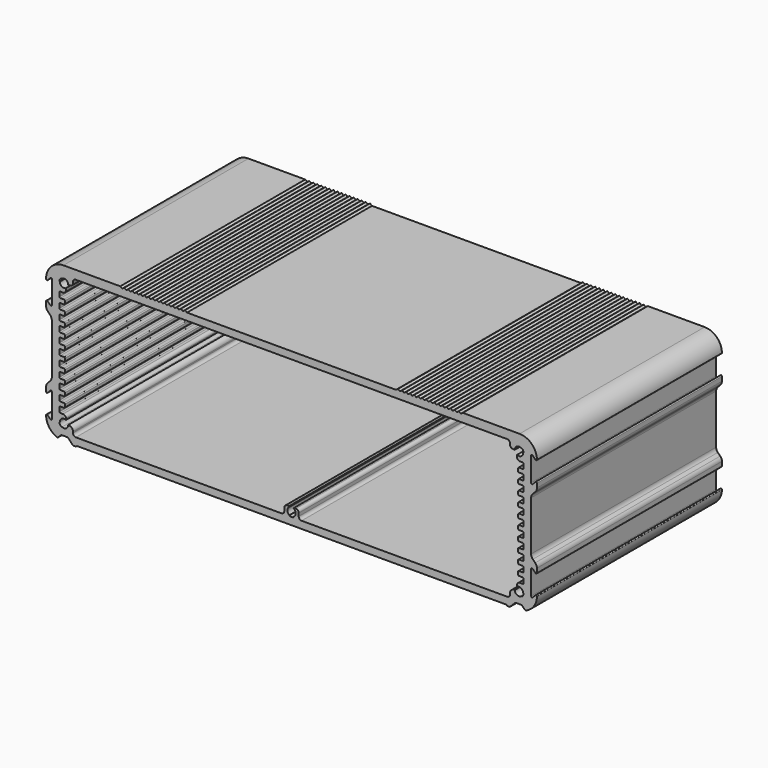
from build123d import *

# Parameters (mm, degrees)
F1_DEPTH = 80


# Not quite as in the source:
# - ends of sketch curves that miss each other by under 0.0002 mm in the source are joined


with BuildPart() as f1:
    # F0 (on Front) → F1 (new body)
    with BuildSketch(Plane.XZ):
        with BuildLine():
            Line((36.15, 26.4), (-36.15, 26.4))
            Line((-36.15, 26.4), (-36.85, 26.9))
            Line((-36.85, 26.9), (-37.55, 26.4))
            Line((-37.55, 26.4), (-38.25, 26.9))
            Line((-38.25, 26.9), (-38.95, 26.4))
            Line((-38.95, 26.4), (-39.65, 26.9))
            Line((-39.65, 26.9), (-40.35, 26.4))
            Line((-40.35, 26.4), (-41.05, 26.9))
            Line((-41.05, 26.9), (-41.75, 26.4))
            Line((-41.75, 26.4), (-42.45, 26.9))
            Line((-42.45, 26.9), (-43.15, 26.4))
            Line((-43.15, 26.4), (-43.85, 26.9))
            Line((-43.85, 26.9), (-44.55, 26.4))
            Line((-44.55, 26.4), (-45.25, 26.9))
            Line((-45.25, 26.9), (-45.95, 26.4))
            Line((-45.95, 26.4), (-46.65, 26.9))
            Line((-46.65, 26.9), (-47.35, 26.4))
            Line((-47.35, 26.4), (-48.05, 26.9))
            Line((-48.05, 26.9), (-48.75, 26.4))
            Line((-48.75, 26.4), (-49.45, 26.9))
            Line((-49.45, 26.9), (-50.15, 26.4))
            Line((-50.15, 26.4), (-50.85, 26.9))
            Line((-50.85, 26.9), (-51.55, 26.4))
            Line((-51.55, 26.4), (-52.25, 26.9))
            Line((-52.25, 26.9), (-52.95, 26.4))
            Line((-52.95, 26.4), (-53.65, 26.9))
            Line((-53.65, 26.9), (-54.35, 26.4))
            Line((-54.35, 26.4), (-55.05, 26.9))
            Line((-55.05, 26.9), (-55.75, 26.4))
            Line((-55.75, 26.4), (-56.45, 26.9))
            Line((-56.45, 26.9), (-57.15, 26.4))
            Line((-57.15, 26.4), (-57.85, 26.9))
            Line((-57.85, 26.9), (-58.55, 26.4))
            Line((-58.55, 26.4), (-59.25, 26.9))
            Line((-59.25, 26.9), (-78.9, 26.9))
            ThreePointArc((-78.9, 26.9), (-83.1426406871, 25.1426406871), (-84.9, 20.9))
            Line((-84.9, 20.9), (-84.9, 20.799264))
            ThreePointArc((-84.9, 20.799264), (-84.7148050297, 20.5221001402), (-84.3878679656, 20.5871319656))
            Line((-84.3878679656, 20.5871319656), (-83.412132, 21.562868))
            ThreePointArc((-83.412132, 21.562868), (-83.0851949703, 21.6278998598), (-82.9, 21.350736))
            Line((-82.9, 21.350736), (-82.9, 13.449264))
            ThreePointArc((-82.9, 13.449264), (-83.0851949703, 13.1721001402), (-83.4121320344, 13.2371319656))
            Line((-83.4121320344, 13.2371319656), (-84.387868, 14.212868))
            ThreePointArc((-84.387868, 14.212868), (-84.7148050297, 14.2778998598), (-84.9, 14.000736))
            Line((-84.9, 14.000736), (-84.9, 12.553427))
            ThreePointArc((-84.9, 12.553427), (-84.7477592003, 11.7880604619), (-84.3142140624, 11.1392139376))
            Line((-84.3142140624, 11.1392139376), (-83.485786, 10.310786))
            ThreePointArc((-83.485786, 10.310786), (-83.0497841884, 9.5556126224), (-82.9000002184, 8.6965730006))
            Line((-82.9000002184, 8.6965730006), (-82.9, -8.396573))
            ThreePointArc((-82.9, -8.396573), (-83.0522407997, -9.1619395381), (-83.4857859376, -9.8107860624))
            Line((-83.4857859376, -9.8107860624), (-84.314214, -10.639214))
            ThreePointArc((-84.314214, -10.639214), (-84.7477592003, -11.2880604619), (-84.9, -12.053427))
            Line((-84.9, -12.053427), (-84.9, -13.500736))
            ThreePointArc((-84.9, -13.500736), (-84.7148050297, -13.7778998598), (-84.3878679656, -13.7128680344))
            Line((-84.3878679656, -13.7128680344), (-83.412132, -12.737132))
            ThreePointArc((-83.412132, -12.737132), (-83.0851949703, -12.6721001402), (-82.9, -12.949264))
            Line((-82.9, -12.949264), (-82.9, -21.250736))
            ThreePointArc((-82.9, -21.250736), (-83.0851949703, -21.5278998598), (-83.4121320344, -21.4628680344))
            Line((-83.4121320344, -21.4628680344), (-84.387868, -20.487132))
            ThreePointArc((-84.387868, -20.487132), (-84.7115889033, -20.4049990304), (-84.8994513764, -20.6811310051))
            ThreePointArc((-84.8994513764, -20.6811310051), (-83.8330713991, -24.0153779543), (-81.0874780686, -26.1870331751))
            ThreePointArc((-81.0874780686, -26.1870331751), (-80.9167083168, -26.2013314216), (-80.7659719656, -26.1198130344))
            Line((-80.7659719656, -26.1198130344), (-79.734027, -25.087868))
            ThreePointArc((-79.734027, -25.087868), (-79.6367000297, -25.0228361402), (-79.521895, -25))
            Line((-79.521895, -25), (-77.575713, -25))
            ThreePointArc((-77.575713, -25), (-77.4609079703, -25.0228361402), (-77.3635809656, -25.0878679656))
            Line((-77.3635809656, -25.0878679656), (-75.551449, -26.9))
            Line((-75.551449, -26.9), (-74.551449, -26.9))
            Line((-74.551449, -26.9), (-74.251449, -26.6))
            Line((-74.251449, -26.6), (74.251449, -26.6))
            Line((74.251449, -26.6), (74.551449, -26.9))
            Line((74.551449, -26.9), (75.551449, -26.9))
            Line((75.551449, -26.9), (77.363581, -25.087868))
            ThreePointArc((77.363581, -25.087868), (77.4609079703, -25.0228361402), (77.575713, -25))
            Line((77.575713, -25), (79.521895, -25))
            ThreePointArc((79.521895, -25), (79.6367000297, -25.0228361402), (79.7340270344, -25.0878679656))
            Line((79.7340270344, -25.0878679656), (80.765972, -26.119813))
            ThreePointArc((80.765972, -26.119813), (80.9167083168, -26.2013314216), (81.0874778713, -26.1870326713))
            ThreePointArc((81.0874778713, -26.1870326713), (83.8330713991, -24.0153779543), (84.8994514549, -20.6811310062))
            ThreePointArc((84.8994514549, -20.6811310062), (84.7115889033, -20.4049990304), (84.3878677463, -20.4871317813))
            Line((84.3878677463, -20.4871317813), (83.412132, -21.462868))
            ThreePointArc((83.412132, -21.462868), (83.0851949703, -21.5278998598), (82.9, -21.250736))
            Line((82.9, -21.250736), (82.9, -12.949264))
            ThreePointArc((82.9, -12.949264), (83.0851949703, -12.6721001402), (83.4121320344, -12.7371319656))
            Line((83.4121320344, -12.7371319656), (84.387868, -13.712868))
            ThreePointArc((84.387868, -13.712868), (84.7148050297, -13.7778998598), (84.9, -13.500736))
            Line((84.9, -13.500736), (84.9, -12.053427))
            ThreePointArc((84.9, -12.053427), (84.7477592003, -11.2880604619), (84.3142140624, -10.6392139376))
            Line((84.3142140624, -10.6392139376), (83.485786, -9.810786))
            ThreePointArc((83.485786, -9.810786), (83.0522407997, -9.1619395381), (82.9, -8.396573))
            Line((82.9, -8.396573), (82.9, 8.696573))
            ThreePointArc((82.9, 8.696573), (83.0522407997, 9.4619395381), (83.4857859376, 10.1107860624))
            Line((83.4857859376, 10.1107860624), (84.314214, 10.939214))
            ThreePointArc((84.314214, 10.939214), (84.7477592003, 11.5880604619), (84.9, 12.353427))
            Line((84.9, 12.353427), (84.9, 13.800736))
            ThreePointArc((84.9, 13.800736), (84.7148050297, 14.0778998598), (84.3878679656, 14.0128680344))
            Line((84.3878679656, 14.0128680344), (83.412132, 13.037132))
            ThreePointArc((83.412132, 13.037132), (83.0851949703, 12.9721001402), (82.9, 13.249264))
            Line((82.9, 13.249264), (82.9, 21.550736))
            ThreePointArc((82.9, 21.550736), (83.0851949703, 21.8278998598), (83.4121320344, 21.7628680344))
            Line((83.4121320344, 21.7628680344), (84.387868, 20.787132))
            ThreePointArc((84.387868, 20.787132), (84.7063723422, 20.7187556671), (84.8994514873, 20.9811309705))
            ThreePointArc((84.8994514873, 20.9811309705), (83.1138589181, 25.171228514), (78.9, 26.9))
            Line((78.9, 26.9), (59.25, 26.9))
            Line((59.25, 26.9), (58.55, 26.4))
            Line((58.55, 26.4), (57.85, 26.9))
            Line((57.85, 26.9), (57.15, 26.4))
            Line((57.15, 26.4), (56.45, 26.9))
            Line((56.45, 26.9), (55.75, 26.4))
            Line((55.75, 26.4), (55.05, 26.9))
            Line((55.05, 26.9), (54.35, 26.4))
            Line((54.35, 26.4), (53.65, 26.9))
            Line((53.65, 26.9), (52.95, 26.4))
            Line((52.95, 26.4), (52.25, 26.9))
            Line((52.25, 26.9), (51.55, 26.4))
            Line((51.55, 26.4), (50.85, 26.9))
            Line((50.85, 26.9), (50.15, 26.4))
            Line((50.15, 26.4), (49.45, 26.9))
            Line((49.45, 26.9), (48.75, 26.4))
            Line((48.75, 26.4), (48.05, 26.9))
            Line((48.05, 26.9), (47.35, 26.4))
            Line((47.35, 26.4), (46.65, 26.9))
            Line((46.65, 26.9), (45.95, 26.4))
            Line((45.95, 26.4), (45.25, 26.9))
            Line((45.25, 26.9), (44.55, 26.4))
            Line((44.55, 26.4), (43.85, 26.9))
            Line((43.85, 26.9), (43.15, 26.4))
            Line((43.15, 26.4), (42.45, 26.9))
            Line((42.45, 26.9), (41.75, 26.4))
            Line((41.75, 26.4), (41.05, 26.9))
            Line((41.05, 26.9), (40.35, 26.4))
            Line((40.35, 26.4), (39.65, 26.9))
            Line((39.65, 26.9), (38.95, 26.4))
            Line((38.95, 26.4), (38.25, 26.9))
            Line((38.25, 26.9), (37.55, 26.4))
            Line((37.55, 26.4), (36.85, 26.9))
            Line((36.85, 26.9), (36.15, 26.4))
        make_face()
        with BuildLine():
            ThreePointArc((-75.6, 22.9), (-75.3071067812, 23.6071067812), (-74.6, 23.9))
            Line((-74.6, 23.9), (74.6, 23.9))
            ThreePointArc((74.6, 23.9), (75.3071067812, 23.6071067812), (75.6, 22.9))
            Line((75.6, 22.9), (75.6, 22.5))
            ThreePointArc((75.6, 22.5), (75.8928932188, 21.7928932188), (76.6, 21.5))
            Line((76.6, 21.5), (77.25, 21.5))
            ThreePointArc((77.25, 21.5), (78.0928837979, 22.8167801324), (79.6415998857, 22.6026738662))
            Line((79.6415998857, 22.6026738662), (79.726192, 22.727571))
            ThreePointArc((79.726192, 22.727571), (80.1494666284, 22.1775296991), (80.3, 21.5))
            Line((80.3, 21.5), (80.15, 21.5))
            ThreePointArc((80.15, 21.5), (79.4497950924, 20.258908819), (78.02543818, 20.2164633425))
            Line((78.02543818, 20.2164633425), (78.025438, 19.520402))
            ThreePointArc((78.025438, 19.520402), (78.3284362903, 18.8325050535), (79.025, 18.55))
            Line((79.025, 18.55), (79.95, 18.55))
            ThreePointArc((79.95, 18.55), (80.1621320344, 18.4621320344), (80.25, 18.25))
            Line((80.25, 18.25), (80.25, 16.85))
            ThreePointArc((80.25, 16.85), (80.1621320344, 16.6378679656), (79.95, 16.55))
            Line((79.95, 16.55), (78.7, 16.55))
            ThreePointArc((78.7, 16.55), (78.4878679656, 16.4621320344), (78.4, 16.25))
            Line((78.4, 16.25), (78.4, 15.35))
            ThreePointArc((78.4, 15.35), (78.4878679656, 15.1378679656), (78.7, 15.05))
            Line((78.7, 15.05), (79.95, 15.05))
            ThreePointArc((79.95, 15.05), (80.1621320344, 14.9621320344), (80.25, 14.75))
            Line((80.25, 14.75), (80.25, 13.35))
            ThreePointArc((80.25, 13.35), (80.1621320344, 13.1378679656), (79.95, 13.05))
            Line((79.95, 13.05), (78.7, 13.05))
            ThreePointArc((78.7, 13.05), (78.4878679656, 12.9621320344), (78.4, 12.75))
            Line((78.4, 12.75), (78.4, 11.85))
            ThreePointArc((78.4, 11.85), (78.4878679656, 11.6378679656), (78.7, 11.55))
            Line((78.7, 11.55), (79.95, 11.55))
            ThreePointArc((79.95, 11.55), (80.1621320344, 11.4621320344), (80.25, 11.25))
            Line((80.25, 11.25), (80.25, 9.85))
            ThreePointArc((80.25, 9.85), (80.1621320344, 9.6378679656), (79.95, 9.55))
            Line((79.95, 9.55), (78.7, 9.55))
            ThreePointArc((78.7, 9.55), (78.4878679656, 9.4621320344), (78.4, 9.25))
            Line((78.4, 9.25), (78.4, 8.35))
            ThreePointArc((78.4, 8.35), (78.4878679656, 8.1378679656), (78.7, 8.05))
            Line((78.7, 8.05), (79.95, 8.05))
            ThreePointArc((79.95, 8.05), (80.1621320344, 7.9621320344), (80.25, 7.75))
            Line((80.25, 7.75), (80.25, 6.35))
            ThreePointArc((80.25, 6.35), (80.1621320344, 6.1378679656), (79.95, 6.05))
            Line((79.95, 6.05), (78.7, 6.05))
            ThreePointArc((78.7, 6.05), (78.4878679656, 5.9621320344), (78.4, 5.75))
            Line((78.4, 5.75), (78.4, 4.85))
            ThreePointArc((78.4, 4.85), (78.4878679656, 4.6378679656), (78.7, 4.55))
            Line((78.7, 4.55), (79.95, 4.55))
            ThreePointArc((79.95, 4.55), (80.1621320344, 4.4621320344), (80.25, 4.25))
            Line((80.25, 4.25), (80.25, 2.85))
            ThreePointArc((80.25, 2.85), (80.1621320344, 2.6378679656), (79.95, 2.55))
            Line((79.95, 2.55), (78.7, 2.55))
            ThreePointArc((78.7, 2.55), (78.4878679656, 2.4621320344), (78.4, 2.25))
            Line((78.4, 2.25), (78.4, 1.35))
            ThreePointArc((78.4, 1.35), (78.4878679656, 1.1378679656), (78.7, 1.05))
            Line((78.7, 1.05), (79.95, 1.05))
            ThreePointArc((79.95, 1.05), (80.1621320344, 0.9621320344), (80.25, 0.75))
            Line((80.25, 0.75), (80.25, -0.65))
            ThreePointArc((80.25, -0.65), (80.1621320344, -0.8621320344), (79.95, -0.95))
            Line((79.95, -0.95), (78.7, -0.95))
            ThreePointArc((78.7, -0.95), (78.4878679656, -1.0378679656), (78.4, -1.25))
            Line((78.4, -1.25), (78.4, -2.15))
            ThreePointArc((78.4, -2.15), (78.4878679656, -2.3621320344), (78.7, -2.45))
            Line((78.7, -2.45), (79.95, -2.45))
            ThreePointArc((79.95, -2.45), (80.1621320344, -2.5378679656), (80.25, -2.75))
            Line((80.25, -2.75), (80.25, -4.15))
            ThreePointArc((80.25, -4.15), (80.1621320344, -4.3621320344), (79.95, -4.45))
            Line((79.95, -4.45), (78.7, -4.45))
            ThreePointArc((78.7, -4.45), (78.4878679656, -4.5378679656), (78.4, -4.75))
            Line((78.4, -4.75), (78.4, -5.65))
            ThreePointArc((78.4, -5.65), (78.4878679656, -5.8621320344), (78.7, -5.95))
            Line((78.7, -5.95), (79.95, -5.95))
            ThreePointArc((79.95, -5.95), (80.1621320344, -6.0378679656), (80.25, -6.25))
            Line((80.25, -6.25), (80.25, -7.65))
            ThreePointArc((80.25, -7.65), (80.1621320344, -7.8621320344), (79.95, -7.95))
            Line((79.95, -7.95), (78.7, -7.95))
            ThreePointArc((78.7, -7.95), (78.4878679656, -8.0378679656), (78.4, -8.25))
            Line((78.4, -8.25), (78.4, -9.15))
            ThreePointArc((78.4, -9.15), (78.4878679656, -9.3621320344), (78.7, -9.45))
            Line((78.7, -9.45), (79.95, -9.45))
            ThreePointArc((79.95, -9.45), (80.1621320344, -9.5378679656), (80.25, -9.75))
            Line((80.25, -9.75), (80.25, -11.15))
            ThreePointArc((80.25, -11.15), (80.1621320344, -11.3621320344), (79.95, -11.45))
            Line((79.95, -11.45), (78.7, -11.45))
            ThreePointArc((78.7, -11.45), (78.4878679656, -11.5378679656), (78.4, -11.75))
            Line((78.4, -11.75), (78.4, -12.65))
            ThreePointArc((78.4, -12.65), (78.4878679656, -12.8621320344), (78.7, -12.95))
            Line((78.7, -12.95), (79.95, -12.95))
            ThreePointArc((79.95, -12.95), (80.1621320344, -13.0378679656), (80.25, -13.25))
            Line((80.25, -13.25), (80.25, -14.65))
            ThreePointArc((80.25, -14.65), (80.1621320344, -14.8621320344), (79.95, -14.95))
            Line((79.95, -14.95), (78.7, -14.95))
            ThreePointArc((78.7, -14.95), (78.4878679656, -15.0378679656), (78.4, -15.25))
            Line((78.4, -15.25), (78.4, -16.15))
            ThreePointArc((78.4, -16.15), (78.4878679656, -16.3621320344), (78.7, -16.45))
            Line((78.7, -16.45), (79.95, -16.45))
            ThreePointArc((79.95, -16.45), (80.1621320344, -16.5378679656), (80.25, -16.75))
            Line((80.25, -16.75), (80.25, -18.15))
            ThreePointArc((80.25, -18.15), (80.1621320344, -18.3621320344), (79.95, -18.45))
            Line((79.95, -18.45), (79.025, -18.45))
            ThreePointArc((79.025, -18.45), (78.3287004935, -18.7322486522), (78.0254601815, -19.4196660055))
            Line((78.0254601815, -19.4196660055), (78.02546, -19.916452))
            ThreePointArc((78.02546, -19.916452), (79.4498056167, -19.9589151773), (80.15, -21.2))
            Line((80.15, -21.2), (80.3, -21.2))
            ThreePointArc((80.3, -21.2), (80.1675788855, -21.8373477973), (79.7922347315, -22.3691977126))
            Line((79.7922347315, -22.3691977126), (79.703775, -22.246392))
            ThreePointArc((79.703775, -22.246392), (78.1312177868, -22.5337866373), (77.25, -21.2))
            Line((77.25, -21.2), (77.1, -21.2))
            ThreePointArc((77.1, -21.2), (76.0393398282, -21.6393398282), (75.6, -22.7))
            Line((75.6, -22.7), (75.6, -23.1))
            ThreePointArc((75.6, -23.1), (75.3071067812, -23.8071067812), (74.6, -24.1))
            Line((74.6, -24.1), (3.5, -24.1))
            ThreePointArc((3.5, -24.1), (2.7928932188, -23.8071067812), (2.5, -23.1))
            Line((2.5, -23.1), (2.5, -22.049445))
            ThreePointArc((2.5, -22.049445), (2.2071067812, -21.3423382188), (1.5, -21.049445))
            Line((1.5, -21.049445), (0.895214, -21.049445))
            ThreePointArc((0.895214, -21.049445), (0.8452139005, -21.0628425171), (0.8086113447, -21.099445199))
            Line((0.8086113447, -21.099445199), (0.725, -21.244263))
            ThreePointArc((0.725, -21.244263), (1.45, -22.5), (0.7249999288, -23.7557368766))
            Line((0.7249999288, -23.7557368766), (0.8, -23.885641))
            ThreePointArc((0.8, -23.885641), (0, -24.1), (-0.7999998467, -23.8856407345))
            Line((-0.7999998467, -23.8856407345), (-0.725, -23.755737))
            ThreePointArc((-0.725, -23.755737), (-1.45, -22.5), (-0.7249999288, -21.2442631234))
            Line((-0.7249999288, -21.2442631234), (-0.808611, -21.099445))
            ThreePointArc((-0.808611, -21.099445), (-0.8452139005, -21.0628425171), (-0.895214, -21.049445))
            Line((-0.895214, -21.049445), (-1.5, -21.049445))
            ThreePointArc((-1.5, -21.049445), (-2.2071067812, -21.3423382188), (-2.5, -22.049445))
            Line((-2.5, -22.049445), (-2.5, -23.1))
            ThreePointArc((-2.5, -23.1), (-2.7928932188, -23.8071067812), (-3.5, -24.1))
            Line((-3.5, -24.1), (-74.6, -24.1))
            ThreePointArc((-74.6, -24.1), (-75.3071067812, -23.8071067812), (-75.6, -23.1))
            Line((-75.6, -23.1), (-75.6, -22.7))
            ThreePointArc((-75.6, -22.7), (-76.0393398282, -21.6393398282), (-77.1, -21.2))
            Line((-77.1, -21.2), (-77.25, -21.2))
            ThreePointArc((-77.25, -21.2), (-77.9501943833, -22.4410848227), (-79.3745400513, -22.4835480977))
            Line((-79.3745400513, -22.4835480977), (-79.44432, -22.616329))
            ThreePointArc((-79.44432, -22.616329), (-80.0694728871, -22.0273717493), (-80.3, -21.2))
            Line((-80.3, -21.2), (-80.15, -21.2))
            ThreePointArc((-80.15, -21.2), (-79.4498056167, -19.9589151773), (-78.0254599487, -19.9164519023))
            Line((-78.0254599487, -19.9164519023), (-78.02546, -19.419666))
            ThreePointArc((-78.02546, -19.419666), (-78.3287004935, -18.7322486522), (-79.025, -18.45))
            Line((-79.025, -18.45), (-79.95, -18.45))
            ThreePointArc((-79.95, -18.45), (-80.1621320344, -18.3621320344), (-80.25, -18.15))
            Line((-80.25, -18.15), (-80.25, -16.75))
            ThreePointArc((-80.25, -16.75), (-80.1621320344, -16.5378679656), (-79.95, -16.45))
            Line((-79.95, -16.45), (-78.7, -16.45))
            ThreePointArc((-78.7, -16.45), (-78.4878679656, -16.3621320344), (-78.4, -16.15))
            Line((-78.4, -16.15), (-78.4, -15.25))
            ThreePointArc((-78.4, -15.25), (-78.4878679656, -15.0378679656), (-78.7, -14.95))
            Line((-78.7, -14.95), (-79.95, -14.95))
            ThreePointArc((-79.95, -14.95), (-80.1621320344, -14.8621320344), (-80.25, -14.65))
            Line((-80.25, -14.65), (-80.25, -13.25))
            ThreePointArc((-80.25, -13.25), (-80.1621320344, -13.0378679656), (-79.95, -12.95))
            Line((-79.95, -12.95), (-78.7, -12.95))
            ThreePointArc((-78.7, -12.95), (-78.4878679656, -12.8621320344), (-78.4, -12.65))
            Line((-78.4, -12.65), (-78.4, -11.75))
            ThreePointArc((-78.4, -11.75), (-78.4878679656, -11.5378679656), (-78.7, -11.45))
            Line((-78.7, -11.45), (-79.95, -11.45))
            ThreePointArc((-79.95, -11.45), (-80.1621320344, -11.3621320344), (-80.25, -11.15))
            Line((-80.25, -11.15), (-80.25, -9.75))
            ThreePointArc((-80.25, -9.75), (-80.1621320344, -9.5378679656), (-79.95, -9.45))
            Line((-79.95, -9.45), (-78.7, -9.45))
            ThreePointArc((-78.7, -9.45), (-78.4878679656, -9.3621320344), (-78.4, -9.15))
            Line((-78.4, -9.15), (-78.4, -8.25))
            ThreePointArc((-78.4, -8.25), (-78.4878679656, -8.0378679656), (-78.7, -7.95))
            Line((-78.7, -7.95), (-79.95, -7.95))
            ThreePointArc((-79.95, -7.95), (-80.1621320344, -7.8621320344), (-80.25, -7.65))
            Line((-80.25, -7.65), (-80.25, -6.25))
            ThreePointArc((-80.25, -6.25), (-80.1621320344, -6.0378679656), (-79.95, -5.95))
            Line((-79.95, -5.95), (-78.7, -5.95))
            ThreePointArc((-78.7, -5.95), (-78.4878679656, -5.8621320344), (-78.4, -5.65))
            Line((-78.4, -5.65), (-78.4, -4.75))
            ThreePointArc((-78.4, -4.75), (-78.4878679656, -4.5378679656), (-78.7, -4.45))
            Line((-78.7, -4.45), (-79.95, -4.45))
            ThreePointArc((-79.95, -4.45), (-80.1621320344, -4.3621320344), (-80.25, -4.15))
            Line((-80.25, -4.15), (-80.25, -2.75))
            ThreePointArc((-80.25, -2.75), (-80.1621320344, -2.5378679656), (-79.95, -2.45))
            Line((-79.95, -2.45), (-78.7, -2.45))
            ThreePointArc((-78.7, -2.45), (-78.4878679656, -2.3621320344), (-78.4, -2.15))
            Line((-78.4, -2.15), (-78.4, -1.25))
            ThreePointArc((-78.4, -1.25), (-78.4878679656, -1.0378679656), (-78.7, -0.95))
            Line((-78.7, -0.95), (-79.95, -0.95))
            ThreePointArc((-79.95, -0.95), (-80.1621320344, -0.8621320344), (-80.25, -0.65))
            Line((-80.25, -0.65), (-80.25, 0.75))
            ThreePointArc((-80.25, 0.75), (-80.1621320344, 0.9621320344), (-79.95, 1.05))
            Line((-79.95, 1.05), (-78.7, 1.05))
            ThreePointArc((-78.7, 1.05), (-78.4878679656, 1.1378679656), (-78.4, 1.35))
            Line((-78.4, 1.35), (-78.4, 2.25))
            ThreePointArc((-78.4, 2.25), (-78.4878679656, 2.4621320344), (-78.7, 2.55))
            Line((-78.7, 2.55), (-79.95, 2.55))
            ThreePointArc((-79.95, 2.55), (-80.1621320344, 2.6378679656), (-80.25, 2.85))
            Line((-80.25, 2.85), (-80.25, 4.25))
            ThreePointArc((-80.25, 4.25), (-80.1621320344, 4.4621320344), (-79.95, 4.55))
            Line((-79.95, 4.55), (-78.7, 4.55))
            ThreePointArc((-78.7, 4.55), (-78.4878679656, 4.6378679656), (-78.4, 4.85))
            Line((-78.4, 4.85), (-78.4, 5.75))
            ThreePointArc((-78.4, 5.75), (-78.4878679656, 5.9621320344), (-78.7, 6.05))
            Line((-78.7, 6.05), (-79.95, 6.05))
            ThreePointArc((-79.95, 6.05), (-80.1621320344, 6.1378679656), (-80.25, 6.35))
            Line((-80.25, 6.35), (-80.25, 7.75))
            ThreePointArc((-80.25, 7.75), (-80.1621320344, 7.9621320344), (-79.95, 8.05))
            Line((-79.95, 8.05), (-78.7, 8.05))
            ThreePointArc((-78.7, 8.05), (-78.4878679656, 8.1378679656), (-78.4, 8.35))
            Line((-78.4, 8.35), (-78.4, 9.25))
            ThreePointArc((-78.4, 9.25), (-78.4878679656, 9.4621320344), (-78.7, 9.55))
            Line((-78.7, 9.55), (-79.95, 9.55))
            ThreePointArc((-79.95, 9.55), (-80.1621320344, 9.6378679656), (-80.25, 9.85))
            Line((-80.25, 9.85), (-80.25, 11.25))
            ThreePointArc((-80.25, 11.25), (-80.1621320344, 11.4621320344), (-79.95, 11.55))
            Line((-79.95, 11.55), (-78.7, 11.55))
            ThreePointArc((-78.7, 11.55), (-78.4878679656, 11.6378679656), (-78.4, 11.85))
            Line((-78.4, 11.85), (-78.4, 12.75))
            ThreePointArc((-78.4, 12.75), (-78.4878679656, 12.9621320344), (-78.7, 13.05))
            Line((-78.7, 13.05), (-79.95, 13.05))
            ThreePointArc((-79.95, 13.05), (-80.1621320344, 13.1378679656), (-80.25, 13.35))
            Line((-80.25, 13.35), (-80.25, 14.75))
            ThreePointArc((-80.25, 14.75), (-80.1621320344, 14.9621320344), (-79.95, 15.05))
            Line((-79.95, 15.05), (-78.7, 15.05))
            ThreePointArc((-78.7, 15.05), (-78.4878679656, 15.1378679656), (-78.4, 15.35))
            Line((-78.4, 15.35), (-78.4, 16.25))
            ThreePointArc((-78.4, 16.25), (-78.4878679656, 16.4621320344), (-78.7, 16.55))
            Line((-78.7, 16.55), (-79.95, 16.55))
            ThreePointArc((-79.95, 16.55), (-80.1621320344, 16.6378679656), (-80.25, 16.85))
            Line((-80.25, 16.85), (-80.25, 18.25))
            ThreePointArc((-80.25, 18.25), (-80.1621320344, 18.4621320344), (-79.95, 18.55))
            Line((-79.95, 18.55), (-79.025, 18.55))
            ThreePointArc((-79.025, 18.55), (-78.3284362903, 18.8325050535), (-78.0254381167, 19.5204020035))
            Line((-78.0254381167, 19.5204020035), (-78.025438, 20.216463))
            ThreePointArc((-78.025438, 20.216463), (-79.4497950924, 20.258908819), (-80.15, 21.5))
            Line((-80.15, 21.5), (-80.3, 21.5))
            ThreePointArc((-80.3, 21.5), (-80.1494666284, 22.1775296991), (-79.7261918836, 22.7275708607))
            Line((-79.7261918836, 22.7275708607), (-79.6416, 22.602674))
            ThreePointArc((-79.6416, 22.602674), (-78.0928837979, 22.8167801324), (-77.25, 21.5))
            Line((-77.25, 21.5), (-76.6, 21.5))
            ThreePointArc((-76.6, 21.5), (-75.8928932188, 21.7928932188), (-75.6, 22.5))
            Line((-75.6, 22.5), (-75.6, 22.9))
        make_face(mode=Mode.SUBTRACT)
    extrude(amount=F1_DEPTH)


solid = f1.part
